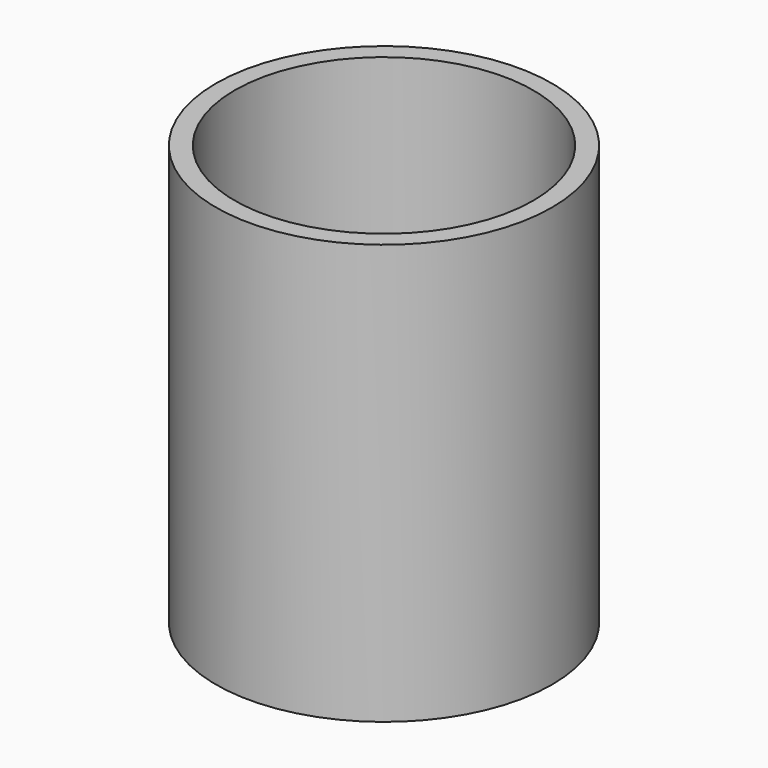
from build123d import *

# Parameters (mm, degrees)
F0_R     = 18
F0_R_2   = 16
F1_DEPTH = 45


# Not quite as in the source:
# - the program builds the solid bodies; features that only make, move or delete a surface that nothing else refers to are left out


with BuildPart() as f1:
    # F0 (on Top) → F1 (new body)
    with BuildSketch(Plane.XY):
        Circle(F0_R)
        Circle(F0_R_2, mode=Mode.SUBTRACT)
    extrude(amount=F1_DEPTH)


solid = f1.part
